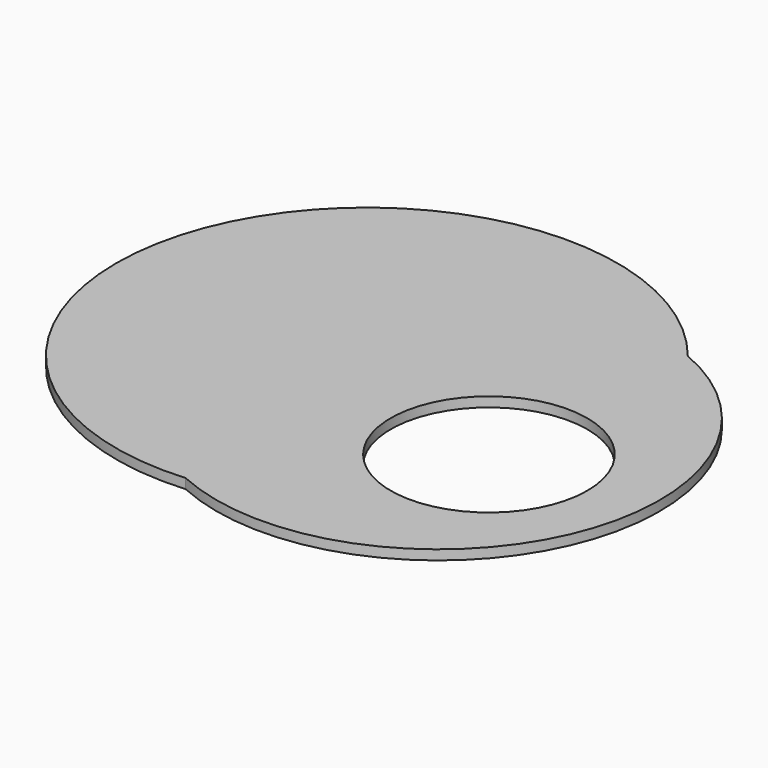
from build123d import *

# Parameters (mm, degrees)
F1_DEPTH = 25.4


with BuildPart() as f1:
    # F0 (on Top) → F1 (new body)
    with BuildSketch(Plane.XY):
        with BuildLine():
            ThreePointArc((5.7862824755, -254.2334721202), (-247.959476671, 93.7900080401), (175.2484512465, 173.8043990925))
            ThreePointArc((175.2484512465, 173.8043990925), (175.3016148465, 178.6025033331), (175.3193363689, 183.4008693695))
            ThreePointArc((175.3193363689, 183.4008693695), (138.9085473628, 397.8323376012), (33.7577623302, 588.2264355431))
            ThreePointArc((33.7577623302, 588.2264355431), (-716.5904978529, 289.2157423962), (-425.9701939676, -464.4219325814))
            ThreePointArc((-425.9701939676, -464.4219325814), (-189.9577330386, -400.6862100109), (5.7862824755, -254.2334721202))
        make_face()
        with BuildLine():
            ThreePointArc((175.3193363689, 183.4008693695), (175.3016148465, 178.6025033331), (175.2484512465, 173.8043990925))
            ThreePointArc((175.2484512465, 173.8043990925), (225.9936293263, 93.404981396), (243.7319752101, 0))
            ThreePointArc((243.7319752101, 0), (174.9658175696, -174.1068716602), (5.7862824755, -254.2334721202))
            ThreePointArc((5.7862824755, -254.2334721202), (-189.9577330386, -400.6862100109), (-425.9701939676, -464.4219325814))
            ThreePointArc((-425.9701939676, -464.4219325814), (121.6131099686, -422.9978230177), (384.131890946, 59.3374558464))
            ThreePointArc((384.131890946, 59.3374558464), (288.592372793, 376.5462131529), (33.7577623302, 588.2264355431))
            ThreePointArc((33.7577623302, 588.2264355431), (138.9085473628, 397.8323376012), (175.3193363689, 183.4008693695))
        make_face()
        with BuildLine():
            ThreePointArc((33.7577623302, 588.2264355431), (-1069.6284842657, 443.399643596), (-425.9701939676, -464.4219325814))
            ThreePointArc((-425.9701939676, -464.4219325814), (-716.5904978529, 289.2157423962), (33.7577623302, 588.2264355431))
        make_face()
    extrude(amount=F1_DEPTH)


solid = f1.part
